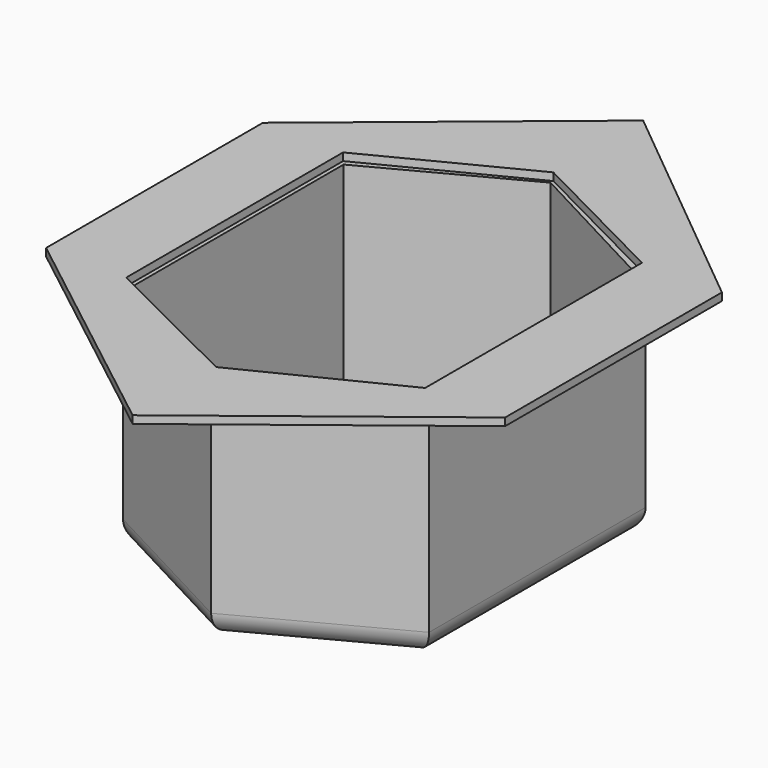
from build123d import *

# Parameters (mm, degrees)
F1_DEPTH = 76.2
F4_DEPTH = 2.54
F5_T     = -2.54
F6_R     = 7.62


# Not quite as in the source:
# - a shell that OpenCascade refuses in one call is made with other operations: the cavity is built on its own and cut out


with BuildPart() as f1:
    # F0 (on Top) → F1 (new body)
    with BuildSketch(Plane.XY):
        Polygon((0, -69.1435125567), (0, 74.5809290344), (-50.8, 47.6656096473), (-50.8, -42.2281931696), align=None)
        Polygon((50.8, 47.6656096473), (0, 74.5809290344), (0, -69.1435125567), (50.8, -42.2281931696), align=None)
    extrude(amount=F1_DEPTH)

    # F3 (on offset) → F4 (join)
    with BuildSketch(Plane.XY.offset(76.2)):
        Polygon((76.2, 47.5584119558), (0, 110.1294793168), (-76.2, 47.5584119558), (-76.2, -42.4090027809), (0, -101.7426550388), (76.2, -42.4090027809), align=None)
        Polygon((-49.5749972761, 47.5584119558), (0, 72.8662833571), (49.6499985456, 47.5584119558), (49.6499985456, -42.4090027809), (0, -67.1015977859), (-49.5749972761, -42.4090027809), align=None, mode=Mode.SUBTRACT)
    extrude(amount=F4_DEPTH)

    # F5: a shell. OpenCascade refuses it in one call, so the cavity is built on its own and cut out:
    # the body offset inwards by the wall thickness, plus a prism from it out through each open face.
    f5_core = offset(f1.part, amount=F5_T, mode=Mode.PRIVATE)
    f5_exits = [f5_core.faces().sort_by_distance(p)[0] for p in [
        (0, 2.718708, 73.66),
    ]]
    add(f5_core, mode=Mode.SUBTRACT)
    extrude(f5_exits, amount=-F5_T, mode=Mode.SUBTRACT)

    # F6
    f6_edges = [f1.edges().sort_by_distance(p)[0] for p in [
        (-25.4, 61.123269, 0),
        (-50.8, 2.718708, 0),
        (-25.4, -55.685853, 0),
        (25.4, -55.685853, 0),
        (50.8, 2.718708, 0),
        (25.4, 61.123269, 0),
    ]]
    fillet(f6_edges, radius=F6_R)


solid = f1.part
